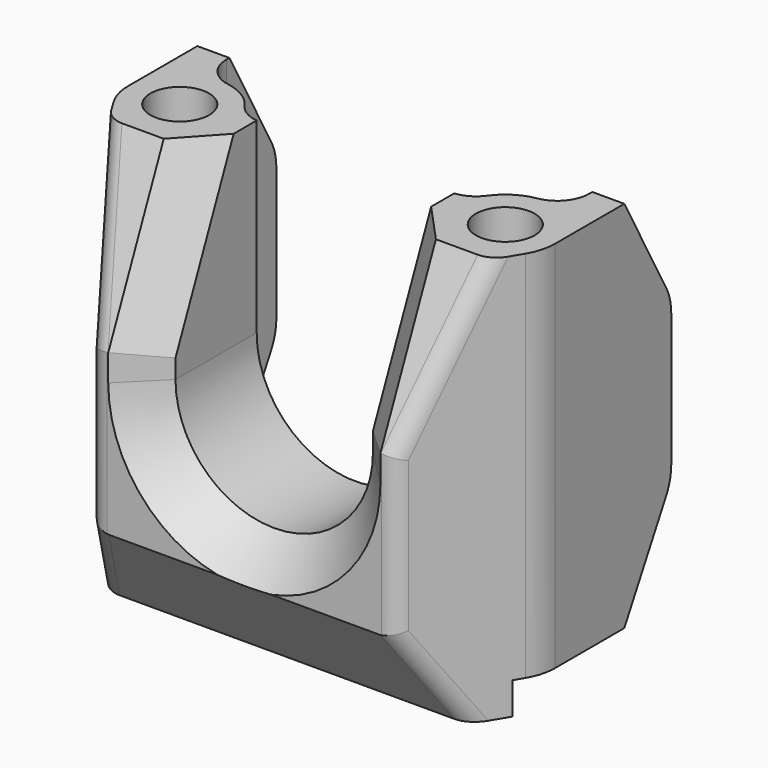
from build123d import *

# Parameters (mm, degrees)
F0_R         = 2.75
F1_DEPTH     = 38
F3_DEPTH     = 3
F5_DEPTH     = 25
F6_SIZE2     = 5
F6_SIZE      = 8
F7_SIZE2     = 6.5
F7_SIZE      = 15
F8_SIZE2     = 6
F8_SIZE      = 10
F9_SIZE2     = 10
F9_SIZE      = 6
F10_R        = 2
F11_C1_SIZE2 = 10
F11_C1_SIZE  = 5.5
F11_C2_SIZE2 = 10
F11_C2_SIZE  = 5.5
F12_SIZE2    = 5.5
F12_SIZE     = 10
F12_2_SIZE2  = 5.5
F12_2_SIZE   = 10
F13_R        = 5
F14_R        = 5
F15_T1_DEPTH = 34.34956364
F15_T3_DEPTH = 11.5008904579
F15_T6_ANGLE = 180


# Not quite as in the source:
# - a fillet or chamfer that OpenCascade refuses, or shapes differently, is made with other operations: its cross-section is extruded or revolved along the edge and cut away or added


with BuildPart() as f1:
    # F0 (on Top) → F1 (new body)
    with BuildSketch(Plane.XY):
        with BuildLine():
            Line((-17, 25), (-20, 25))
            Line((-20, 25), (-20, 0))
            Line((-20, 0), (20, 0))
            Line((20, 0), (20, 25))
            Line((20, 25), (17, 25))
            Line((17, 25), (17, 19.1485292704))
            ThreePointArc((17, 19.1485292704), (16.286002286, 17.205800893), (14.4838709677, 16.1878082625))
            ThreePointArc((14.4838709677, 16.1878082625), (12.7404153064, 15.5329250756), (11.3827554868, 14.2580645161))
            ThreePointArc((11.3827554868, 14.2580645161), (10.3140016776, 13.332997333), (8.9402852679, 13))
            Line((8.9402852679, 13), (-8.9402852679, 13))
            ThreePointArc((-8.9402852679, 13), (-10.3140016776, 13.332997333), (-11.3827554868, 14.2580645161))
            ThreePointArc((-11.3827554868, 14.2580645161), (-12.7404153064, 15.5329250756), (-14.4838709677, 16.1878082625))
            ThreePointArc((-14.4838709677, 16.1878082625), (-16.286002286, 17.205800893), (-17, 19.1485292704))
            Line((-17, 19.1485292704), (-17, 25))
        make_face()
        with Locations((-15.25, 11.5)):
            Circle(F0_R, mode=Mode.SUBTRACT)
        with Locations((15.25, 11.5)):
            Circle(F0_R, mode=Mode.SUBTRACT)
    extrude(amount=F1_DEPTH)

    # F2 (on face) → F3 (cut)
    with BuildSketch(Plane(origin=(0, 0, 0), x_dir=(1, 0, 0), z_dir=(0, 0, -1))):
        with BuildLine():
            Line((18, -7.8), (-18, -7.8))
            ThreePointArc((-18, -7.8), (-19.4142135624, -8.3857864376), (-20, -9.8))
            Line((-20, -9.8), (-20, -60))
            Line((-20, -60), (20, -60))
            Line((20, -60), (20, -9.8))
            ThreePointArc((20, -9.8), (19.4142135624, -8.3857864376), (18, -7.8))
        make_face()
    extrude(amount=-F3_DEPTH, mode=Mode.SUBTRACT)

    # F4 (on face) → F5 (cut)
    with BuildSketch(Plane.XZ):
        with BuildLine():
            Line((-9.25, 38), (-9.25, 20.5))
            ThreePointArc((-9.25, 20.5), (0, 11.25), (9.25, 20.5))
            Line((9.25, 20.5), (9.25, 38))
            Line((9.25, 38), (-9.25, 38))
        make_face()
    extrude(amount=-F5_DEPTH, mode=Mode.SUBTRACT)

    # F6
    f6_edges = [f1.edges().sort_by_distance(p)[0] for p in [
        (0, 0, 0),
    ]]
    f6_side = f1.faces().sort_by_distance((0, 0, 0.551725))[0]
    chamfer(f6_edges, length=F6_SIZE, length2=F6_SIZE2, reference=f6_side)

    # F7
    f7_edges = [f1.edges().sort_by_distance(p)[0] for p in [
        (-14.625, 0, 38),
        (14.625, 0, 38),
    ]]
    f7_side = f1.faces().sort_by_distance((19.5, 0, 23))[0]
    chamfer(f7_edges, length=F7_SIZE, length2=F7_SIZE2, reference=f7_side)

    # F8
    f8_edges = [f1.edges().sort_by_distance(p)[0] for p in [
        (20, 0, 15.5),
    ]]
    f8_side = f1.faces().sort_by_distance((20, 13.094719, 19.529129))[0]
    chamfer(f8_edges, length=F8_SIZE, length2=F8_SIZE2, reference=f8_side)

    # F9
    f9_edges = [f1.edges().sort_by_distance(p)[0] for p in [
        (-20, 0, 15.5),
    ]]
    f9_side = f1.faces().sort_by_distance((11.625, 0, 22.628382))[0]
    chamfer(f9_edges, length=F9_SIZE, length2=F9_SIZE2, reference=f9_side)

    # F10
    f10_edges = [f1.edges().sort_by_distance(p)[0] for p in [
        (15.95, 3.25, 30.5),
        (-15.95, 3.25, 30.5),
        (14, 0, 15.5),
        (-14, 0, 15.5),
        (-15.5, 2.5, 4),
        (15.5, 2.5, 4),
    ]]
    fillet(f10_edges, radius=F10_R)

    # F11: chamfer of 10 x 5.5 on 2 edges, made by hand

    # F11_c1
    f11_c1_edges = [f1.edges().sort_by_distance(p)[0] for p in [
        (-18.5, 25, 3),
    ]]
    f11_c1_side = f1.faces().sort_by_distance((-18.5, 24.89, 3))[0]
    chamfer(f11_c1_edges, length=F11_C1_SIZE, length2=F11_C1_SIZE2, reference=f11_c1_side)

    # F11_c2
    f11_c2_edges = [f1.edges().sort_by_distance(p)[0] for p in [
        (18.5, 25, 3),
    ]]
    f11_c2_side = f1.faces().sort_by_distance((18.5, 24.89, 3))[0]
    chamfer(f11_c2_edges, length=F11_C2_SIZE, length2=F11_C2_SIZE2, reference=f11_c2_side)

    # F12
    f12_edges = [f1.edges().sort_by_distance(p)[0] for p in [
        (18.5, 25, 38),
    ]]
    f12_side = f1.faces().sort_by_distance((18.5, 25, 25.5))[0]
    chamfer(f12_edges, length=F12_SIZE, length2=F12_SIZE2, reference=f12_side)

    # F12#2
    f12_2_edges = [f1.edges().sort_by_distance(p)[0] for p in [
        (-18.5, 25, 38),
    ]]
    f12_2_side = f1.faces().sort_by_distance((-18.5, 25, 25.5))[0]
    chamfer(f12_2_edges, length=F12_2_SIZE, length2=F12_2_SIZE2, reference=f12_2_side)

    # F13
    f13_edges = [f1.edges().sort_by_distance(p)[0] for p in [
        (20, 10, 20.5),
        (-20, 10, 20.5),
    ]]
    fillet(f13_edges, radius=F13_R)

    # F14
    f14_edges = [f1.edges().sort_by_distance(p)[0] for p in [
        (18.5, 25, 28),
        (18.5, 25, 13),
        (-18.5, 25, 13),
        (-18.5, 25, 28),
    ]]
    fillet(f14_edges, radius=F14_R)

    # F15: chamfer of 3.5 on 5 edges, made by hand

    # F15_s2 → F15_t1 (cut)
    with BuildSketch(Plane(origin=(0, 4.8121986531, 11.1050738149), x_dir=(1, 0, 0), z_dir=(0, 0.3976074376, 0.9175556253))):
        Polygon((-12.75, -9.1449710656), (-9.25, -5.6449710656), (-9.25, -9.1449710656), align=None)
        Polygon((9.25, -5.6449710656), (12.75, -9.1449710656), (9.25, -9.1449710656), align=None)
    extrude(amount=F15_T1_DEPTH, mode=Mode.SUBTRACT)

    # F15_s4 → F15_t3 (cut)
    with BuildSketch(Plane.XY.offset(20.5)):
        Polygon((-9.25, 3.5), (-12.75, 0), (-9.25, 0), align=None)
        Polygon((12.75, 0), (9.25, 3.5), (9.25, 0), align=None)
    extrude(amount=F15_T3_DEPTH, mode=Mode.SUBTRACT)

    # F15_s5 → F15_t6 (revolve, cut)
    with BuildSketch(Plane.XY.offset(20.5)):
        Polygon((-12.75, 0), (-9.25, 3.5), (-9.25, 0), align=None)
    revolve(axis=Axis((0, 0, 20.5), (0, -1, 0)), revolution_arc=F15_T6_ANGLE, mode=Mode.SUBTRACT)


solid = f1.part
